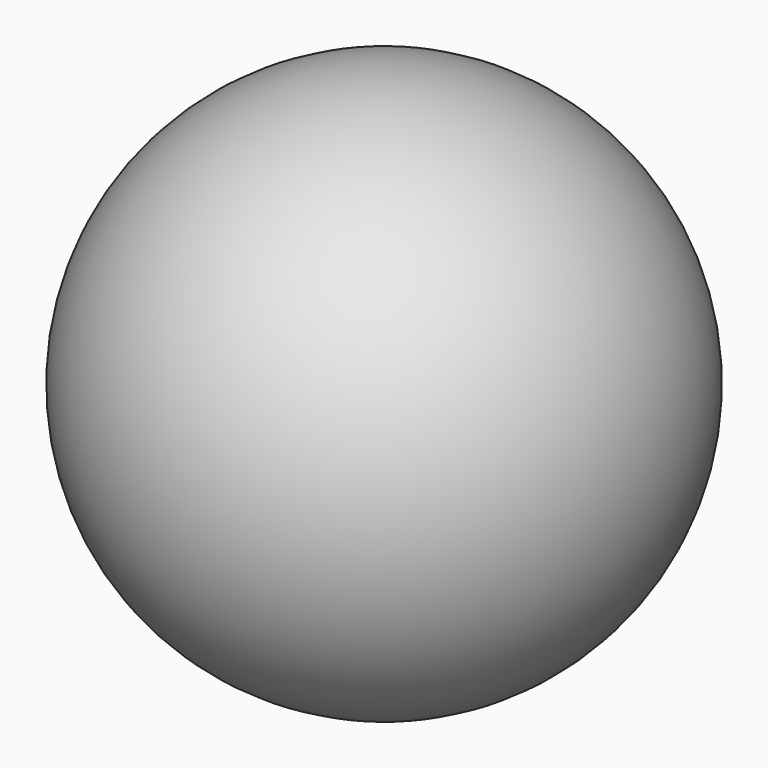
from build123d import *

# Parameters (mm, degrees)
F4_SIZE = 1


# Not quite as in the source:
# - a fillet or chamfer that OpenCascade refuses, or shapes differently, is made with other operations: its cross-section is extruded or revolved along the edge and cut away or added


with BuildPart() as f1:
    # F0 (on Front) → F1 (revolve)
    with BuildSketch(Plane.XZ):
        with BuildLine():
            Line((0, 28), (0, 35))
            ThreePointArc((0, 35), (-17.3691143388, 19.6363209229), (-4.2406859855, 0.5215848098))
            Line((-4.2406859855, 0.5215848098), (-3.75, 28))
            Line((-3.75, 28), (0, 28))
        make_face()
    revolve(axis=Axis((0, 0, 16.7157072574), (0, 0, -1)))

    # F2: chamfer of 0.5 x 3 on 1 edges, made by hand

    # F2_s1 → F2_t2 (revolve, cut)
    with BuildSketch(Plane.XZ):
        with BuildLine():
            Line((-4.1607847025, 3.6471133949), (-4.8506659959, 0.5610496404))
            Line((-4.8506659959, 0.5610496404), (-4.8672070924, 0.5033747574))
            ThreePointArc((-4.8672070924, 0.5033747574), (-4.5463653864, 0.5387452771), (-4.2552254803, 0.4633731005))
            Line((-4.2552254803, 0.4633731005), (-4.1806955496, 0.520513552))
            ThreePointArc((-4.1806955496, 0.520513552), (-4.152785205, 2.0834928499), (-4.1007942666, 3.6460421371))
            Line((-4.1007942666, 3.6460421371), (-4.1607847025, 3.6471133949))
        make_face()
    revolve(axis=Axis((0, 0, 0.5215848098), (0, 0, -1)), mode=Mode.SUBTRACT)

    # F4
    f4_edges = [f1.edges().sort_by_distance(p)[0] for p in [
        (3.75, 0, 28),
    ]]
    chamfer(f4_edges, length=F4_SIZE)


solid = f1.part
